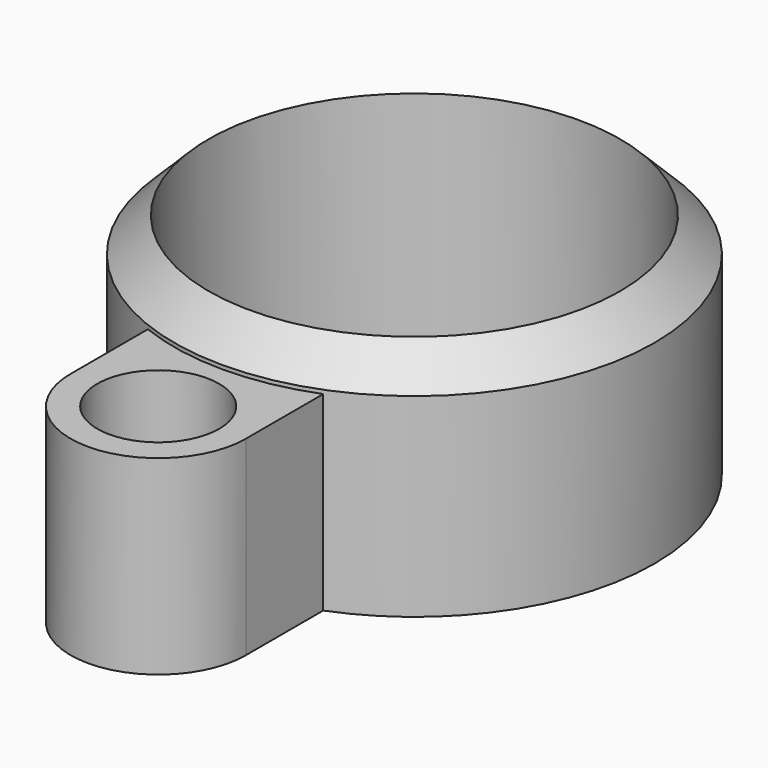
from build123d import *

# Parameters (mm, degrees)
F0_R     = 8.001
F0_R_2   = 6.858
F1_DEPTH = 7.747
F3_R     = 2.032
F4_DEPTH = 6.35


# Not quite as in the source:
# - a fillet or chamfer that OpenCascade refuses, or shapes differently, is made with other operations: its cross-section is extruded or revolved along the edge and cut away or added


with BuildPart() as f1:
    # F0 (on Top) → F1 (new body)
    with BuildSketch(Plane.XY):
        Circle(F0_R)
        Circle(F0_R_2, mode=Mode.SUBTRACT)
    extrude(amount=F1_DEPTH)

    # F2: chamfer of 1.27 on 1 edges, made by hand

    # F2_s1 → F2_t2 (revolve, cut)
    with BuildSketch(Plane.XZ):
        Polygon((8.001, 6.477), (6.731, 7.747), (8.001, 7.747), align=None)
    revolve(axis=Axis((0, 0, 7.747), (0, 0, 1)), mode=Mode.SUBTRACT)

    # F3 (on face) → F4 (join)
    with BuildSketch(Plane(origin=(0, 0, 0), x_dir=(1, 0, 0), z_dir=(0, 0, -1))):
        with BuildLine():
            Line((2.921, 7.4487421757), (2.921, 10.668))
            ThreePointArc((2.921, 10.668), (0, 13.589), (-2.921, 10.668))
            Line((-2.921, 10.668), (-2.921, 7.4487421757))
            ThreePointArc((-2.921, 7.4487421757), (0, 8.001), (2.921, 7.4487421757))
        make_face()
        with Locations((0, 10.668)):
            Circle(F3_R, mode=Mode.SUBTRACT)
    extrude(amount=-F4_DEPTH)


solid = f1.part
